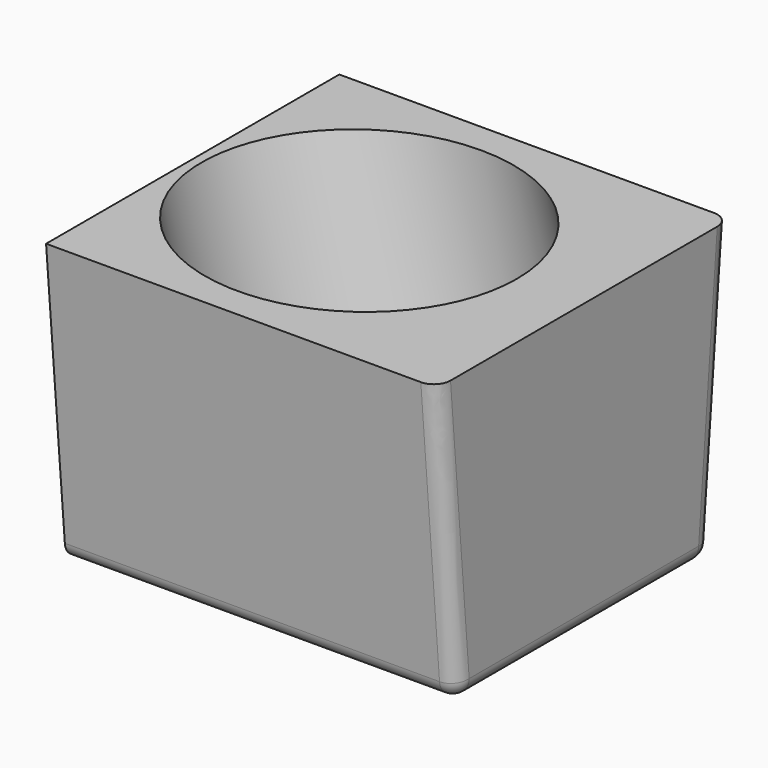
from build123d import *

# Parameters (mm, degrees)
F2_W     = 95
F2_H     = 89
F0_W     = 95
F0_H     = 77
F7_R     = 37
F8_DEPTH = 85.8
F9_R     = 4


# Not quite as in the source:
# - a feature names something its author has since deleted; it is built from what else it names


with BuildPart() as f3:
    # F2 (on offset) → F3 section 0
    with BuildSketch(Plane.XY.offset(70)):
        with Locations((-47.5, -38.5)):
            Rectangle(F2_W, F2_H)
    # F0 (on Top) → F3 section 1
    with BuildSketch(Plane.XY):
        with Locations((-47.5, -38.5)):
            Rectangle(F0_W, F0_H)
    loft()

    # F7 (on face) → F8 (cut)
    with BuildSketch(Plane(origin=(-27.2627936506, 0, 102.6103478024), x_dir=(0.966468953, 0, 0.2567834941), z_dir=(-0.2567834941, 0, 0.966468953))):
        with Locations((-34.7436182201, -38.5)):
            Circle(F7_R)
    extrude(amount=-F8_DEPTH, mode=Mode.SUBTRACT)

    # F9
    f9_edges = [f3.edges().sort_by_distance(p)[0] for p in [
        (-47.5, -77, 0),
        (0, -38.5, 0),
        (-47.5, 0, 0),
        (0, -80, 35),
        (0, 3, 35),
    ]]
    fillet(f9_edges, radius=F9_R)


solid = f3.part
